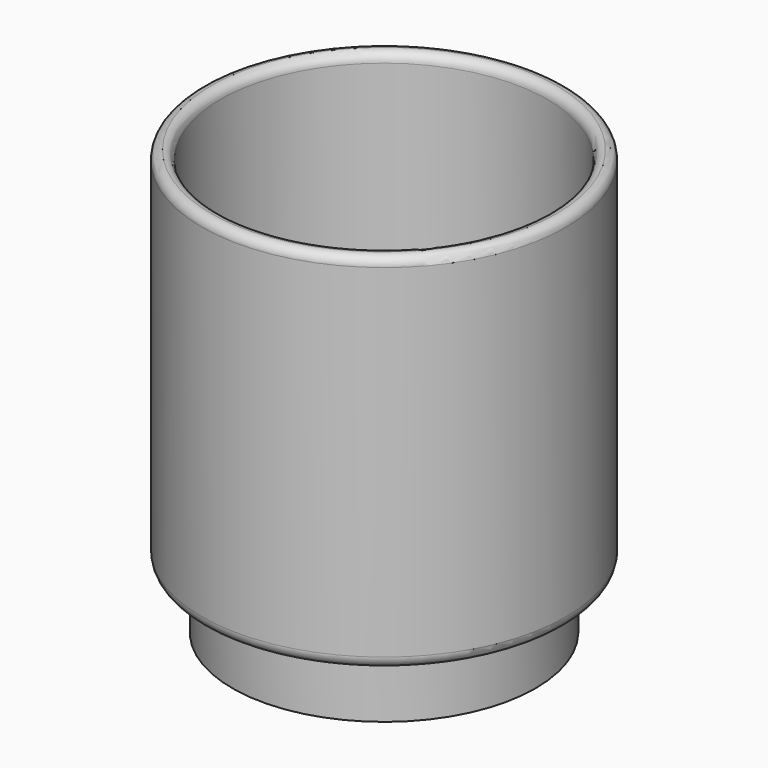
from build123d import *

# Parameters (mm, degrees)
F0_R       = 30
F1_DEPTH   = 60
F2_R       = 27
F1_FACE1_R = 30
F3_DEPTH   = 55
F4_R       = 25
F5_DEPTH   = 10
F6_R       = 20
F7_DEPTH   = 10
F8_R       = 1.49999
F9_R       = 2
F10_R      = 2


# Not quite as in the source:
# - a fillet or chamfer is up to 0.001 mm smaller than in the source, because OpenCascade refuses the exact size


with BuildPart() as f1:
    # F0 (on Top) → F1 (new body)
    with BuildSketch(Plane.XY):
        Circle(F0_R)
    extrude(amount=F1_DEPTH)

    # F2 (on face) + F1_face1 (on face) → F3 (cut)
    with BuildSketch(Plane.XY.offset(60)):
        Circle(F2_R)
    with BuildSketch(Plane(origin=(0, 0, 0), x_dir=(1, 0, 0), z_dir=(0, 0, -1))):
        Circle(F1_FACE1_R)
    extrude(amount=-F3_DEPTH, dir=(0, 0, 1), mode=Mode.SUBTRACT)

    # F4 (on face) → F5 (join)
    with BuildSketch(Plane(origin=(0, 0, 0), x_dir=(1, 0, 0), z_dir=(0, 0, -1))):
        Circle(F4_R)
    extrude(amount=F5_DEPTH)

    # F6 (on face) → F7 (cut)
    with BuildSketch(Plane(origin=(0, 0, -10), x_dir=(1, 0, 0), z_dir=(0, 0, -1))):
        Circle(F6_R)
    extrude(amount=-F7_DEPTH, mode=Mode.SUBTRACT)

    # F8 (radius 1.5 in the source; OpenCascade refuses exactly that, so slightly less here)
    f8_edges = [f1.edges().sort_by_distance(p)[0] for p in [
        (-30, 0, 60),
        (-27, 0, 60),
    ]]
    fillet(f8_edges, radius=F8_R)

    # F9
    f9_edges = [f1.edges().sort_by_distance(p)[0] for p in [
        (-30, 0, 0),
    ]]
    fillet(f9_edges, radius=F9_R)

    # F10
    f10_edges = [f1.edges().sort_by_distance(p)[0] for p in [
        (-27, 0, 5),
    ]]
    fillet(f10_edges, radius=F10_R)


solid = f1.part
